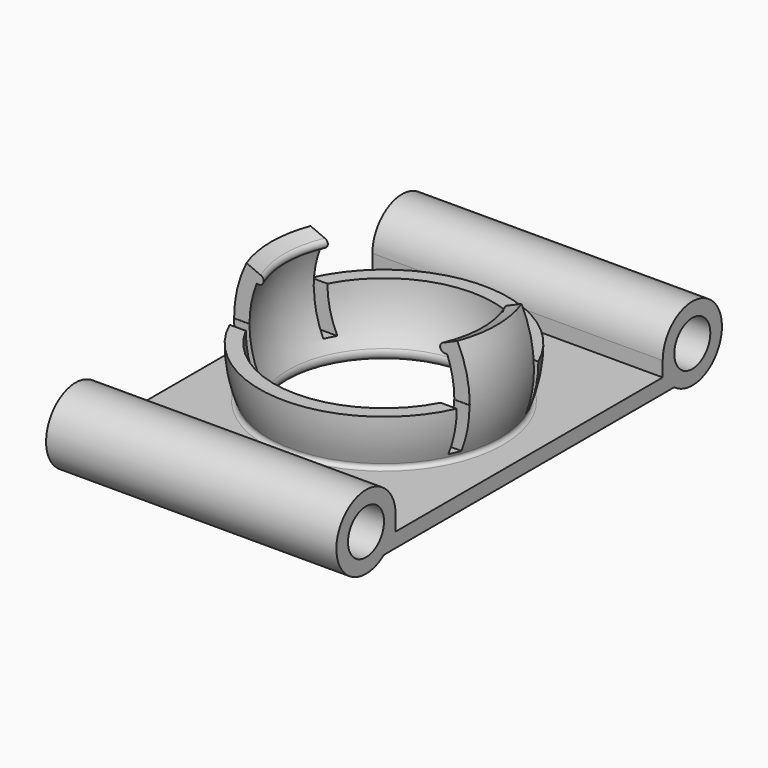
from build123d import *

# Parameters (mm, degrees)
F4_W      = 37.3510532081
F4_H      = 13.2476640865
F5_DEPTH  = 25
F6_W      = 1.474830322
F6_H      = 5.8938292786
F7_DEPTH  = 25
F9_DEPTH  = 2
F10_R     = 3.1
F11_DEPTH = 40


# Not quite as in the source:
# - a pattern or mirror of a feature is missing from the dataset's text; its kind, count and spacing are read off the source's solid
# - the program builds the solid bodies; features that only make, move or delete a surface that nothing else refers to are left out


with BuildPart() as f3:
    # F2 (on Front) → F3 (revolve)
    with BuildSketch(Plane.XZ):
        with BuildLine():
            Line((-13.7305629736, 6.4026666654), (-15.5431785477, 7.2479031889))
            ThreePointArc((-15.5431785477, 7.2479031889), (-17.1424918778, 0.5074172037), (-15.9446656173, -6.3158640227))
            ThreePointArc((-15.9446656173, -6.3158640227), (-15.9959621092, -6.7810089067), (-16.4095246732, -7))
            Line((-16.4095246732, -7), (-20, -7))
            Line((-20, -7), (-20, -9))
            Line((-20, -9), (-14.029344247, -9))
            ThreePointArc((-14.029344247, -9), (-13.164660479, -8.5023166147), (-13.1606542007, -7.5046439628))
            ThreePointArc((-13.1606542007, -7.5046439628), (-15.0974297932, -1.2609970819), (-14.2232523076, 5.217431724))
            ThreePointArc((-14.2232523076, 5.217431724), (-13.3967149096, 5.5688693575), (-13.7305629736, 6.4026666654))
        make_face()
    revolve(axis=Axis((0, 0, -2.5768550113), (0, 0, 1)))

    # F4 (on Top) → F5 (cut)
    with BuildSketch(Plane.XY):
        with Locations((-0.0919979066, 12.1436924674)):
            Rectangle(F4_W, F4_H)
    f5 = extrude(amount=F5_DEPTH, mode=Mode.SUBTRACT)

    # F5_copies: F5 across plane
    add(f5.mirror(Plane(origin=(0, 0, 0), x_dir=(0, 0, -1), z_dir=(0, -1, 0))), mode=Mode.SUBTRACT)

    # F6 (on Right) → F7 (cut, symmetric)
    with BuildSketch(Plane.YZ):
        with Locations((-6.29051961, -2.9469146393)):
            Rectangle(F6_W, F6_H)
    f7 = extrude(amount=F7_DEPTH, both=True, mode=Mode.SUBTRACT)

    # F7_copies: F7 across plane
    add(f7.mirror(Plane.ZX), mode=Mode.SUBTRACT)

    # F8 (on face) → F9 (join)
    with BuildSketch(Plane(origin=(0, 0, -9), x_dir=(1, 0, 0), z_dir=(0, 0, -1))):
        with BuildLine():
            Line((20, 0), (20, 25))
            Line((20, 25), (-20, 25))
            Line((-20, 25), (-20, 0))
            ThreePointArc((-20, 0), (0, 20), (20, 0))
        make_face()
        with BuildLine():
            Line((20, -25), (20, 0))
            ThreePointArc((20, 0), (0, -20), (-20, 0))
            Line((-20, 0), (-20, -25))
            Line((-20, -25), (20, -25))
        make_face()
    extrude(amount=-F9_DEPTH)

    # F10 (on face) → F11 (join)
    with BuildSketch(Plane.YZ.offset(20)):
        with BuildLine():
            Line((23, -7), (25, -7))
            Line((25, -7), (25, -9))
            ThreePointArc((25, -9), (32.6727453461, -2.6919906956), (23, -4.9503086537))
            Line((23, -4.9503086537), (23, -7))
        make_face()
        with Locations((28.1, -4.9503086537)):
            Circle(F10_R, mode=Mode.SUBTRACT)
    f11 = extrude(amount=-F11_DEPTH)

    # F11_copies: F11 across plane
    add(f11.mirror(Plane(origin=(0, 0, 0), x_dir=(0, 0, -1), z_dir=(0, -1, 0))))


solid = f3.part
